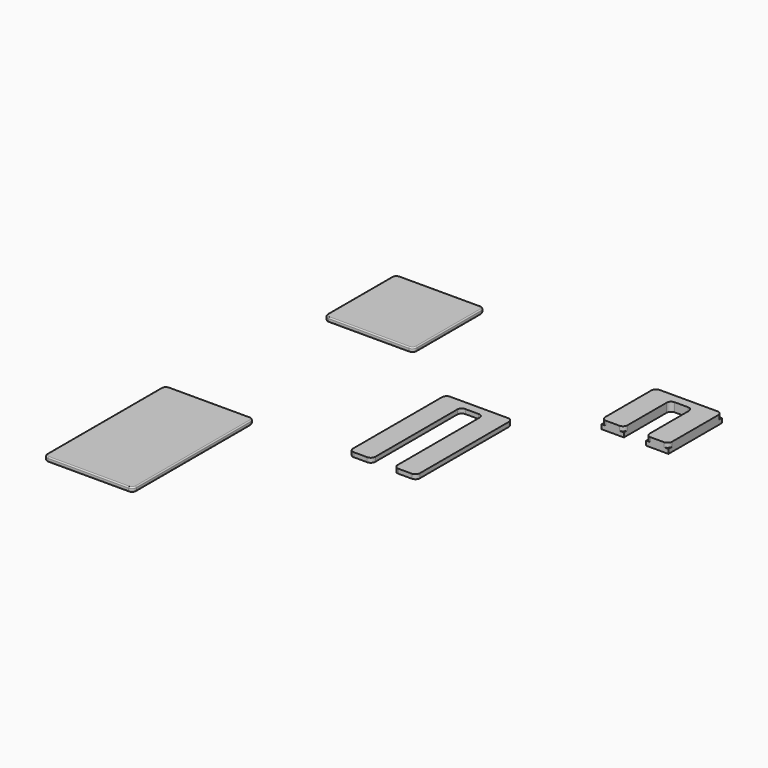
from build123d import *

# Parameters (mm, degrees)
F0_W      = 20
F0_H      = 20
F1_DEPTH  = 1
F2_R      = 1
F3_R      = 0.25
F5_DEPTH  = 2
F6_R      = 1
F8_DEPTH  = 1
F9_R      = 1
F10_W     = 20
F10_H     = 34
F11_DEPTH = 1
F12_R     = 1
F13_R     = 0.25
F14_R     = 1


# Not quite as in the source:
# - two fillets or chamfers of one size are made in one step


with BuildPart() as f1:
    # F0 (on Top) → F1 (new body)
    with BuildSketch(Plane.XY):
        with Locations((-32.9304196417, 40.2150040078)):
            Rectangle(F0_W, F0_H)
    extrude(amount=F1_DEPTH)

    # F2
    f2_edges = [f1.edges().sort_by_distance(p)[0] for p in [
        (-42.93042, 50.215004, 0.5),
        (-22.93042, 50.215004, 0.5),
        (-22.93042, 30.215004, 0.5),
        (-42.93042, 30.215004, 0.5),
    ]]
    fillet(f2_edges, radius=F2_R)

    # F3
    f3_edges = [f1.edges().sort_by_distance(p)[0] for p in [
        (-32.93042, 30.215004, 1),
        (-22.93042, 40.215004, 0),
        (-22.93042, 31.215004, 0.5),
        (-22.93042, 49.215004, 0.5),
        (-22.93042, 40.215004, 1),
    ]]
    fillet(f3_edges, radius=F3_R)


with BuildPart() as f5:
    # F4 (on Top) → F5 (new body)
    with BuildSketch(Plane.XY):
        Polygon((35.7377539144, 43.4313830447), (20.7377539144, 43.4313830447), (20.7377539144, 28.4313830447), (25.7377539144, 28.4313830447), (25.7377539144, 41.4313830447), (30.7377539144, 41.4313830447), (30.7377539144, 28.4313830447), (35.7377539144, 28.4313830447), align=None)
    extrude(amount=F5_DEPTH)

    # F6
    f6_edges = [f5.edges().sort_by_distance(p)[0] for p in [
        (35.737754, 43.431383, 1),
        (20.737754, 43.431383, 1),
        (35.737754, 28.431383, 1),
        (30.737754, 28.431383, 1),
        (25.737754, 28.431383, 1),
        (20.737754, 28.431383, 1),
        (25.737754, 41.431383, 1),
        (30.737754, 41.431383, 1),
    ]]
    fillet(f6_edges, radius=F6_R)

    # F4 (on Top) → F8 (join)
    with BuildSketch(Plane.XY):
        Polygon((35.7377539144, 43.4313830447), (20.7377539144, 43.4313830447), (20.7377539144, 28.4313830447), (25.7377539144, 28.4313830447), (25.7377539144, 41.4313830447), (30.7377539144, 41.4313830447), (30.7377539144, 28.4313830447), (35.7377539144, 28.4313830447), align=None)
    extrude(amount=F8_DEPTH)


with BuildPart() as f8:
    # F4 (on Top) → F8, piece 2 (new body)
    with BuildSketch(Plane.XY):
        Polygon((7.5, 20), (-7.5, 20), (-7.5, -7), (-2.5, -7), (-2.5, 18), (2.5, 18), (2.5, -7), (7.5, -7), align=None)
    extrude(amount=F8_DEPTH)

    # F9
    f9_edges = [f8.edges().sort_by_distance(p)[0] for p in [
        (-7.5, -7, 0.5),
        (2.5, -7, 0.5),
        (-2.5, -7, 0.5),
        (7.5, -7, 0.5),
        (7.5, 20, 0.5),
        (-7.5, 20, 0.5),
    ]]
    fillet(f9_edges, radius=F9_R)

    # F14
    f14_edges = [f8.edges().sort_by_distance(p)[0] for p in [
        (-2.5, 18, 0.5),
        (2.5, 18, 0.5),
    ]]
    fillet(f14_edges, radius=F14_R)


with BuildPart() as f11:
    # F10 (on Top) → F11 (new body)
    with BuildSketch(Plane.XY):
        with Locations((-38.1617667153, -24.8989770475)):
            Rectangle(F10_W, F10_H)
    extrude(amount=F11_DEPTH)

    # F12
    f12_edges = [f11.edges().sort_by_distance(p)[0] for p in [
        (-28.161767, -41.898977, 0.5),
        (-28.161767, -7.898977, 0.5),
        (-48.161767, -41.898977, 0.5),
        (-48.161767, -7.898977, 0.5),
    ]]
    fillet(f12_edges, radius=F12_R)

    # F13
    f13_edges = [f11.edges().sort_by_distance(p)[0] for p in [
        (-28.161767, -24.898977, 1),
        (-28.45466, -41.606084, 1),
        (-28.45466, -8.19187, 1),
        (-38.161767, -41.898977, 1),
        (-38.161767, -7.898977, 1),
        (-47.868873, -41.606084, 1),
        (-47.868873, -8.19187, 1),
        (-48.161767, -24.898977, 1),
        (-28.161767, -24.898977, 0),
        (-28.45466, -41.606084, 0),
        (-28.45466, -8.19187, 0),
        (-38.161767, -41.898977, 0),
        (-38.161767, -7.898977, 0),
        (-47.868873, -41.606084, 0),
        (-47.868873, -8.19187, 0),
        (-48.161767, -24.898977, 0),
    ]]
    fillet(f13_edges, radius=F13_R)


solid = Compound([f1.part, f5.part, f8.part, f11.part])
